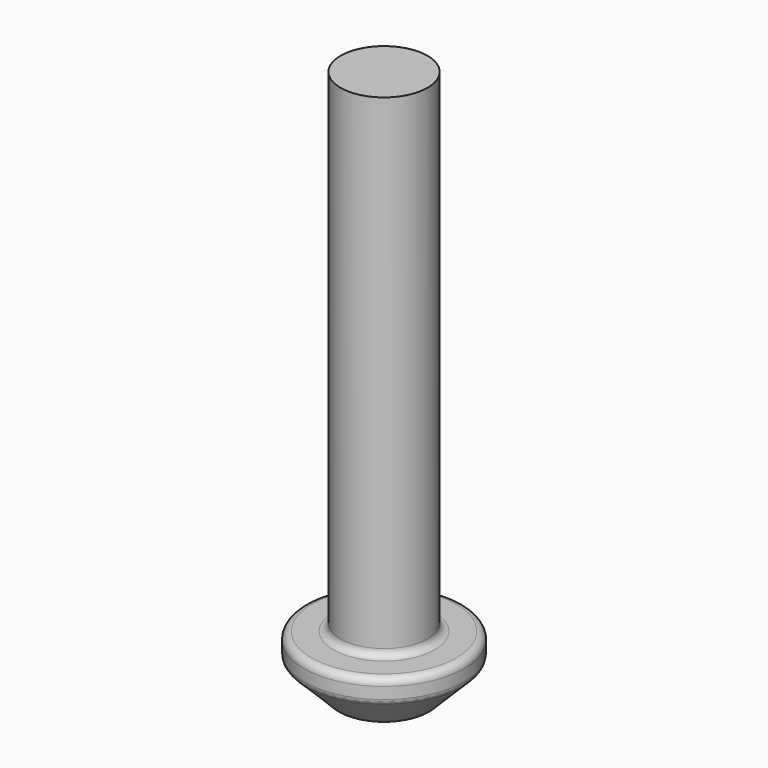
from build123d import *

# Parameters (mm, degrees)
F1_R     = 2.75
F1_R_2   = 1.5
F2_DEPTH = 2
F3_START = 1.5
F3_DEPTH = 0.5
F4_START = 2
F4_DEPTH = 17
F5_SIZE2 = 1.25
F5_SIZE  = 1.25
F6_R     = 0.25


# Not quite as in the source:
# - a feature names something its author has since deleted; it is built from what else it names


with BuildPart() as f2:
    # F1 (on Top) → F2 (new body)
    with BuildSketch(Plane.XY):
        Circle(F1_R)
        Circle(F1_R_2, mode=Mode.SUBTRACT)
        Circle(F1_R_2)
        Polygon((-0.5773502692, -1), (-1.1547005384, 0), (-0.5773502692, 1), (0.5773502692, 1), (1.1547005384, 0), (0.5773502692, -1), align=None, mode=Mode.SUBTRACT)
    extrude(amount=F2_DEPTH)

    # F1 (on Top) → F3 (join)
    with BuildSketch(Plane.XY.offset(F3_START)):
        Polygon((-0.5773502692, 1), (-1.1547005384, 0), (-0.5773502692, -1), (0.5773502692, -1), (1.1547005384, 0), (0.5773502692, 1), align=None)
    extrude(amount=F3_DEPTH)

    # F1 (on Top) → F4 (join)
    with BuildSketch(Plane.XY.offset(F4_START)):
        Circle(F1_R_2)
        Polygon((-0.5773502692, -1), (-1.1547005384, 0), (-0.5773502692, 1), (0.5773502692, 1), (1.1547005384, 0), (0.5773502692, -1), align=None, mode=Mode.SUBTRACT)
        Polygon((-0.5773502692, 1), (-1.1547005384, 0), (-0.5773502692, -1), (0.5773502692, -1), (1.1547005384, 0), (0.5773502692, 1), align=None)
    extrude(amount=F4_DEPTH)

    # F5
    f5_edges = [f2.edges().sort_by_distance(p)[0] for p in [
        (-2.75, 0, 0),
    ]]
    chamfer(f5_edges, length=F5_SIZE, length2=F5_SIZE2)

    # F6
    f6_edges = [f2.edges().sort_by_distance(p)[0] for p in [
        (-2.75, 0, 2),
        (-1.5, 0, 2),
        (-1.5, 0, 0),
        (-2.75, 0, 1.25),
    ]]
    fillet(f6_edges, radius=F6_R)


solid = f2.part
